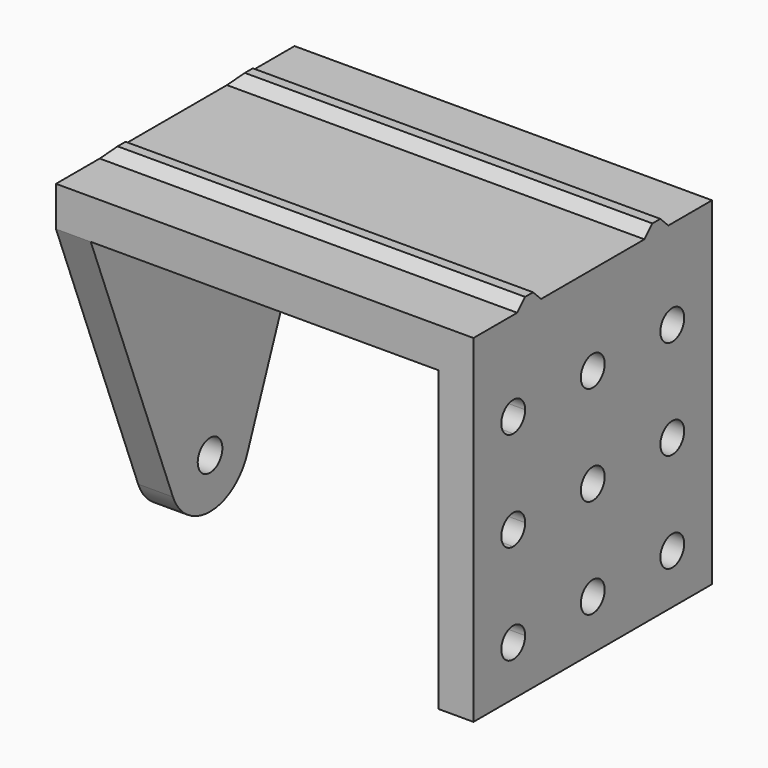
from build123d import *

# Parameters (mm, degrees)
F0_W          = 42
F0_H          = 30
F1_DEPTH      = 4
F2_W          = 3.5
F2_H          = 30
F3_DEPTH      = 30
F4_R          = 1.55
F5_DEPTH      = 5
F7_DEPTH      = 3.5
F8_W          = 42
F8_H          = 4
F9_DEPTH      = 1
F10_SIZE      = 1
F11_T4_DEPTH  = 48.7150489639
F11_T9_DEPTH  = 48.7150489639
F11_T14_DEPTH = 48.7150489639
F11_T19_DEPTH = 48.7150489639
F12_R         = 1.5
F13_DEPTH     = 3.5


# Not quite as in the source:
# - a fillet or chamfer that OpenCascade refuses, or shapes differently, is made with other operations: its cross-section is extruded or revolved along the edge and cut away or added


with BuildPart() as f1:
    # F0 (on Top) → F1 (new body)
    with BuildSketch(Plane.XY):
        Rectangle(F0_W, F0_H)
    extrude(amount=F1_DEPTH)

    # F2 (on face) → F3 (join)
    with BuildSketch(Plane(origin=(0, 0, 0), x_dir=(1, 0, 0), z_dir=(0, 0, -1))):
        with Locations((-19.25, 0)):
            Rectangle(F2_W, F2_H)
        with Locations((19.25, 0)):
            Rectangle(F2_W, F2_H)
    extrude(amount=F3_DEPTH)

    # F4 (on face) → F5 (cut)
    with BuildSketch(Plane(origin=(-21, 0, 0), x_dir=(0, -1, 0), z_dir=(-1, 0, 0))):
        with Locations((0, -25)):
            Circle(F4_R)
    extrude(amount=-F5_DEPTH, mode=Mode.SUBTRACT)

    # F6 (on face) → F7 (cut)
    with BuildSketch(Plane(origin=(-21, 0, 0), x_dir=(0, -1, 0), z_dir=(-1, 0, 0))):
        with BuildLine():
            ThreePointArc((0, -30), (-2.8288373248, -29.1228242007), (-4.665119593, -26.7990717558))
            Line((-4.665119593, -26.7990717558), (-15, 0))
            Line((-15, 0), (-15, -30))
            Line((-15, -30), (0, -30))
        make_face()
        with BuildLine():
            ThreePointArc((4.665119593, -26.7990717558), (2.8288373248, -29.1228242007), (0, -30))
            Line((0, -30), (15, -30))
            Line((15, -30), (15, 0))
            Line((15, 0), (4.665119593, -26.7990717558))
        make_face()
    extrude(amount=-F7_DEPTH, mode=Mode.SUBTRACT)

    # F8 (on face) → F9 (join)
    with BuildSketch(Plane.XY.offset(4)):
        with Locations((0, 8)):
            Rectangle(F8_W, F8_H)
        with Locations((0, -8)):
            Rectangle(F8_W, F8_H)
    extrude(amount=F9_DEPTH)

    # F10
    f10_edges = [f1.edges().sort_by_distance(p)[0] for p in [
        (-21, -8, 5),
        (-21, 8, 5),
    ]]
    chamfer(f10_edges, length=F10_SIZE)

    # F11: chamfer of 1.5 on 4 edges, made by hand


with BuildPart() as f11_tool2:
    # F11_s3 → F11_t4 (new body)
    with BuildSketch(Plane.YZ.offset(-23.8575244819)):
        Polygon((-8.5, 5), (-10, 3.5), (-10, 5), align=None)
    extrude(amount=F11_T4_DEPTH)

    split(bisect_by=Plane.XY.offset(4), keep=Keep.TOP)


with BuildPart() as f1_1:
    add(f1.part)

    # F11_t1: cut F11_tool2
    add(f11_tool2.part, mode=Mode.SUBTRACT)


with BuildPart() as f11_tool7:
    # F11_s8 → F11_t9 (new body)
    with BuildSketch(Plane.YZ.offset(24.8575244819)):
        Polygon((-6, 3.5), (-7.5, 5), (-6, 5), align=None)
    extrude(amount=-F11_T9_DEPTH)

    split(bisect_by=Plane.XY.offset(4), keep=Keep.TOP)


with BuildPart() as f1_2:
    add(f1_1.part)

    # F11_t6: cut F11_tool7
    add(f11_tool7.part, mode=Mode.SUBTRACT)


with BuildPart() as f11_tool12:
    # F11_s13 → F11_t14 (new body)
    with BuildSketch(Plane.YZ.offset(-23.8575244819)):
        Polygon((6, 3.5), (7.5, 5), (6, 5), align=None)
    extrude(amount=F11_T14_DEPTH)

    split(bisect_by=Plane.XY.offset(4), keep=Keep.TOP)


with BuildPart() as f1_3:
    add(f1_2.part)

    # F11_t11: cut F11_tool12
    add(f11_tool12.part, mode=Mode.SUBTRACT)


with BuildPart() as f11_tool17:
    # F11_s18 → F11_t19 (new body)
    with BuildSketch(Plane.YZ.offset(24.8575244819)):
        Polygon((10, 3.5), (8.5, 5), (10, 5), align=None)
    extrude(amount=-F11_T19_DEPTH)

    split(bisect_by=Plane.XY.offset(4), keep=Keep.TOP)


with BuildPart() as f1_4:
    add(f1_3.part)

    # F11_t16: cut F11_tool17
    add(f11_tool17.part, mode=Mode.SUBTRACT)

    # F12 (on face) → F13 (cut)
    with BuildSketch(Plane.YZ.offset(21)):
        with BuildLine():
            ThreePointArc((-10, -6.5), (-8.9393398282, -6.0606601718), (-8.5, -5))
            ThreePointArc((-8.5, -5), (-11.0606601718, -3.9393398282), (-10, -6.5))
        make_face()
        with BuildLine():
            ThreePointArc((-8.5, -25), (-8.9393398282, -23.9393398282), (-10, -23.5))
            ThreePointArc((-10, -23.5), (-11.0606601718, -26.0606601718), (-8.5, -25))
        make_face()
        with BuildLine():
            ThreePointArc((-8.5, -15), (-8.9393398282, -13.9393398282), (-10, -13.5))
            Line((-10, -13.5), (-10, -16.5))
            ThreePointArc((-10, -16.5), (-8.9393398282, -16.0606601718), (-8.5, -15))
        make_face()
        with BuildLine():
            Line((-10, -16.5), (-10, -13.5))
            ThreePointArc((-10, -13.5), (-11.5, -15), (-10, -16.5))
        make_face()
        with Locations((0, -5)):
            Circle(F12_R)
        with Locations((10, -5)):
            Circle(F12_R)
        with Locations((0, -15)):
            Circle(F12_R)
        with Locations((0, -25)):
            Circle(F12_R)
        with Locations((10, -15)):
            Circle(F12_R)
        with Locations((10, -25)):
            Circle(F12_R)
    extrude(amount=-F13_DEPTH, mode=Mode.SUBTRACT)


solid = f1_4.part
